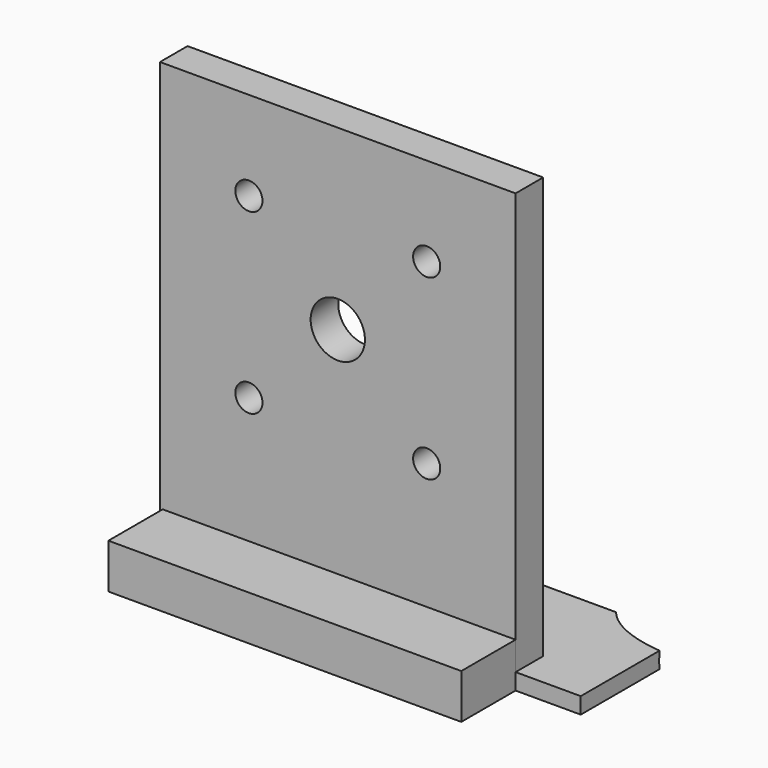
from build123d import *
from build123d import SkipClean  # not in build123d's __all__

# Parameters (mm, degrees)
F0_W      = 131
F0_H      = 155.25
F0_R      = 5
F0_R_2    = 10
F1_DEPTH  = 12.7
F2_DEPTH  = 150
F3_R      = 4.7625
F4_DEPTH  = 167.951
F6_DEPTH  = 55
F9_W      = 46.4503765106
F9_H      = 23.6088857055
F10_DEPTH = 100.6187200546
F12_DEPTH = 150.001
F14_DEPTH = 89.0000760555
F15_R     = 18.8692896997
F16_DEPTH = 210.4837932836
F18_W     = 28.0103459954
F18_H     = 33.3821959794
F19_DEPTH = 57.4413500726
F23_DEPTH = 37.3063087463
F25_DEPTH = 262.8513174901
F26_W     = 130
F26_H     = 33
F27_DEPTH = 25
F28_DEPTH = 47.1665114164
F29_W     = 130
F29_H     = 16.5
F30_DEPTH = 374.0004003048


with BuildPart() as f1:
    # F0 (on Front) → F1 (new body)
    with BuildSketch(Plane.XZ):
        with Locations((0, 77.625)):
            Rectangle(F0_W, F0_H)
        with Locations((-32.75, 57)):
            Circle(F0_R, mode=Mode.SUBTRACT)
        with Locations((32.75, 57)):
            Circle(F0_R, mode=Mode.SUBTRACT)
        with Locations((0, 89.75)):
            Circle(F0_R_2, mode=Mode.SUBTRACT)
        with Locations((-32.75, 122.5)):
            Circle(F0_R, mode=Mode.SUBTRACT)
        with Locations((32.75, 122.5)):
            Circle(F0_R, mode=Mode.SUBTRACT)
    extrude(amount=-F1_DEPTH)

    # F0 (on Front) → F2 (join)
    with BuildSketch(Plane.XZ):
        Polygon((89.5, 0), (65.5, 0), (-65.5, 0), (-65.5, -12.7), (89.5, -12.7), align=None)
    extrude(amount=-F2_DEPTH)

    # F3 (on face) → F4 (cut, through all)
    with BuildSketch(Plane(origin=(0, 0, -12.7), x_dir=(1, 0, 0), z_dir=(0, 0, -1))):
        with Locations((-40, -55.7)):
            Circle(F3_R)
        with Locations((-40, -118.2)):
            Circle(F3_R)
        with Locations((64, -118.2)):
            Circle(F3_R)
        with Locations((64, -55.7)):
            Circle(F3_R)
    extrude(amount=-F4_DEPTH, mode=Mode.SUBTRACT)

    # F5 (on face) → F6 (join)
    with BuildSketch(Plane.XZ):
        Polygon((76.5, -12.7), (-63.5, -12.7), (-44.9285714286, -100.7630571853), align=None)
    extrude(amount=-F6_DEPTH)

    # F7 (on face) → F8 (revolve)
    with BuildSketch(Plane(origin=(32.4031609217, 0, -44.6801379177), x_dir=(0.8095238095, 0, 0.5870870479), z_dir=(0.5870870479, 0, -0.8095238095))):
        Polygon((18.2698592544, -37.5), (54.4725659202, -37.5), (54.4725659202, -30), (-45.5274340798, -30), (-45.5274340798, -37.5), align=None)
    revolve(axis=Axis((36.0238095238, 55, -42.0543523951), (-0.8095238095, 0, -0.5870870479)))

    # F9 (on face) → F10 (cut)
    with BuildSketch(Plane.YZ.offset(89.5)):
        with Locations((57.3695674539, 11.8044428527)):
            Rectangle(F9_W, F9_H)
    extrude(amount=-F10_DEPTH, mode=Mode.SUBTRACT)

    # F11 (on Front) → F12 (cut, through all)
    with BuildSketch(Plane.XZ):
        Polygon((-55.6169226766, -72.8361010551), (-44.6262694895, -72.8361010551), (-44.6262694895, -12.6905664802), (-63.8953074813, -12.6905664802), (-63.8953074813, -72.8361010551), align=None)
        Polygon((-4.5890193433, -104.113265872), (-4.5890193433, -72.8361010551), (-44.6262694895, -72.8361010551), (-55.6169226766, -72.8361010551), (-55.6169226766, -104.113265872), align=None)
    extrude(amount=-F12_DEPTH, mode=Mode.SUBTRACT)

    # F13 (on face) → F14 (cut)
    with BuildSketch(Plane(origin=(0, 55, 0), x_dir=(-1, 0, 0), z_dir=(0, 1, 0))):
        Polygon((76.3912552581, -71.6465198879), (44.6262694895, -60.2878452083), (44.6262694895, -72.8361010551), (6.4205920826, -72.8361010551), (4.4523809524, -71.4087047902), (-10.0519139283, -91.4084170785), (37.2047263411, -125.6801223738), align=None)
        Polygon((44.6262694895, -60.2878452083), (19.1295571499, -51.1706095521), (14.7264042907, -57.2420381235), (4.4523809524, -71.4087047902), (6.4205920826, -72.8361010551), (44.6262694895, -72.8361010551), align=None)
    extrude(amount=-F14_DEPTH, mode=Mode.SUBTRACT)

    # F15 (on face) → F16 (cut, through all)
    with BuildSketch(Plane(origin=(-36.8555418741, 0, -26.7285668724), x_dir=(0, -1, 0), z_dir=(-0.8095238095, 0, -0.5870870479))):
        with Locations((-55, -55.1931115454)):
            Circle(F15_R)
        with BuildLine():
            ThreePointArc((-37.5, -55.1931115454), (-67.3743686708, -67.5674802162), (-55, -37.6931115454))
            Line((-55, -37.6931115454), (-55, -55.1931115454))
            Line((-55, -55.1931115454), (-37.5, -55.1931115454))
        make_face(mode=Mode.SUBTRACT)
        with BuildLine():
            Line((-55, -55.1931115454), (-55, -37.6931115454))
            ThreePointArc((-55, -37.6931115454), (-67.3743686708, -67.5674802162), (-37.5, -55.1931115454))
            Line((-37.5, -55.1931115454), (-55, -55.1931115454))
        make_face()
    with SkipClean():  # cleaning this boolean's faces spoils the solid; the shape is the same uncleaned
        extrude(amount=-F16_DEPTH, mode=Mode.SUBTRACT)

    # F18 (on offset) → F19 (cut)
    with BuildSketch(Plane(origin=(0, 0, -69.7121929049), x_dir=(1, 0, 0), z_dir=(0, 0, -1))):
        with Locations((-40.2482412755, -55.8588486165)):
            Rectangle(F18_W, F18_H)
    with SkipClean():  # cleaning this boolean's faces spoils the solid; the shape is the same uncleaned
        extrude(amount=-F19_DEPTH, mode=Mode.SUBTRACT)

    # F22 (on offset) → F23 (join)
    with BuildSketch(Plane(origin=(0, 66.3563400507, 0), x_dir=(-1, 0, 0), z_dir=(0, 1, 0))):
        Polygon((-19.5, -25.368578732), (9.2864632607, -47.1396760544), (25.5, -47.1396760544), (25.5, -10.8354373375), (-19.5, -10.8354373375), align=None)
    with SkipClean():  # cleaning this boolean's faces spoils the solid; the shape is the same uncleaned
        extrude(amount=-F23_DEPTH)

    # F24 (on offset) → F25 (cut, through all)
    with BuildSketch(Plane(origin=(0, 0, -107.6003174901), x_dir=(1, 0, 0), z_dir=(0, 0, -1))):
        Polygon((105.054743588, -47.2050309181), (-70.2532827854, -47.2050309181), (-70.2532827854, -164.4858419895), (108.5324063897, -164.4858419895), align=None)
    extrude(amount=-F25_DEPTH, mode=Mode.SUBTRACT)

    # F26 (on Front) → F27 (join)
    with BuildSketch(Plane.XZ):
        with Locations((0.4943662184, -6)):
            Rectangle(F26_W, F26_H)
    extrude(amount=F27_DEPTH)

    # F28 (add): a face of the model
    f28_faces = [f1.faces().sort_by_distance(p)[0] for p in [
        (-54.5656671683, 0, -17.5954279167),
    ]]
    extrude(f28_faces, amount=F28_DEPTH)

    # F29 (on face) → F30 (cut)
    with BuildSketch(Plane.XZ.offset(25)):
        Polygon((102.4388783057, -90.8307954669), (102.4388783057, -6), (65.4943662184, -6), (65.4943662184, -22.5), (-64.5056337816, -22.5), (-64.5056337816, -6), (-95.0750373681, -6), (-96.5073853731, -90.8307954669), align=None)
        with Locations((0.4943662184, -14.25)):
            Rectangle(F29_W, F29_H)
    extrude(amount=-F30_DEPTH, mode=Mode.SUBTRACT)


solid = f1.part
